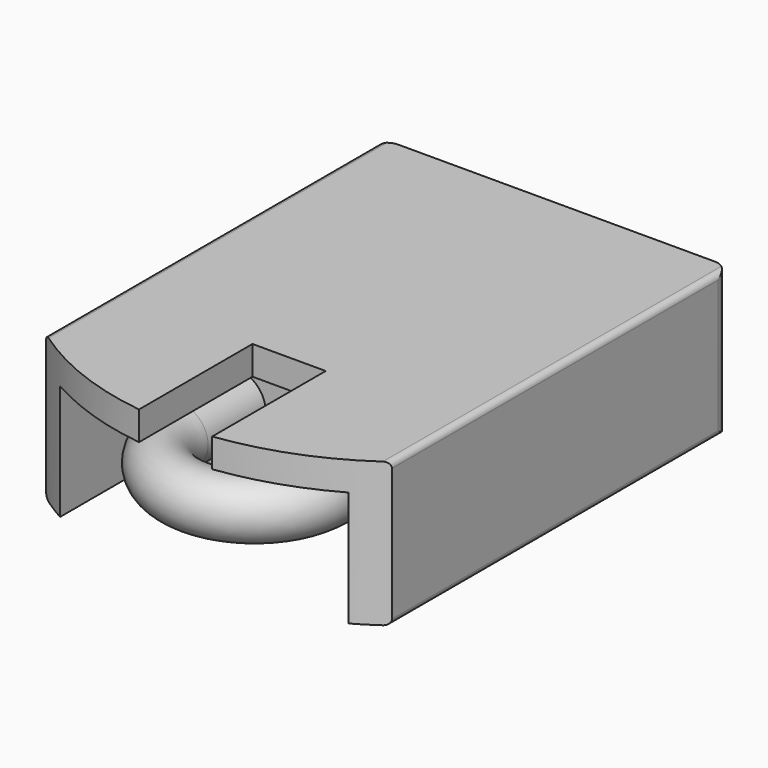
from build123d import *

# Parameters (mm, degrees)
F1_DEPTH    = 25
F3_R        = 2.54
F4_W        = 50
F4_H        = 30
F5_DEPTH    = 20
F2_W        = 12.7
F2_H        = 25
F6_DEPTH    = 25
F7_T1_DEPTH = 75.655609521
F9_W        = 5
F9_H        = 15
F10_DEPTH   = 10
F11_W       = 7.3
F11_H       = 11.5
F12_DEPTH   = 25.4
F15_R       = 4.9651178244


# Not quite as in the source:
# - a fillet or chamfer that OpenCascade refuses, or shapes differently, is made with other operations: its cross-section is extruded or revolved along the edge and cut away or added
# - a feature names something its author has since deleted; it is built from what else it names


with BuildPart() as f1:
    # F0 (on Top) → F1 (new body)
    with BuildSketch(Plane.XY):
        with BuildLine():
            Line((30, -36.5978047605), (30, 36.5978047605))
            Line((30, 36.5978047605), (-30, 36.5978047605))
            Line((-30, 36.5978047605), (-30, -36.5978047605))
            ThreePointArc((-30, -36.5978047605), (0, -46.4021952395), (30, -36.5978047605))
        make_face()
    extrude(amount=F1_DEPTH)

    # F3
    f3_edges = [f1.edges().sort_by_distance(p)[0] for p in [
        (-30, 36.597805, 12.5),
        (30, 36.597805, 12.5),
    ]]
    fillet(f3_edges, radius=F3_R)

    # F4 (on face) → F5 (cut)
    with BuildSketch(Plane.XY):
        with Locations((0, -31.4021952395)):
            Rectangle(F4_W, F4_H)
    extrude(amount=F5_DEPTH, mode=Mode.SUBTRACT)

    # F2 (on Top) → F6 (cut, through all)
    with BuildSketch(Plane.XY):
        with Locations((0, -33.9021952395)):
            Rectangle(F2_W, F2_H)
    extrude(amount=F6_DEPTH, mode=Mode.SUBTRACT)

    # F7: fillet of radius 1 on 4 edges, made by hand

    # F7_s2 → F7_t1 (cut)
    with BuildSketch(Plane.XZ.offset(-36.5578047605)):
        with BuildLine():
            ThreePointArc((29, 0), (29.7071067812, 0.2928932188), (30, 1))
            Line((30, 1), (30, 0))
            Line((30, 0), (29, 0))
        make_face()
        with BuildLine():
            ThreePointArc((29, 25), (29.7071067812, 24.7071067812), (30, 24))
            Line((30, 24), (30, 25))
            Line((30, 25), (29, 25))
        make_face()
        with BuildLine():
            ThreePointArc((-29, 25), (-29.7071067812, 24.7071067812), (-30, 24))
            Line((-30, 24), (-30, 25))
            Line((-30, 25), (-29, 25))
        make_face()
        with BuildLine():
            ThreePointArc((-29, 0), (-29.7071067812, 0.2928932188), (-30, 1))
            Line((-30, 1), (-30, 0))
            Line((-30, 0), (-29, 0))
        make_face()
    extrude(amount=F7_T1_DEPTH, mode=Mode.SUBTRACT)

    # F9 (on face) → F10 (cut)
    with BuildSketch(Plane(origin=(0, 36.5978047605, 0), x_dir=(-1, 0, 0), z_dir=(0, 1, 0))):
        with Locations((-15.5, 12.5)):
            Rectangle(F9_W, F9_H)
        with Locations((15.5, 12.5)):
            Rectangle(F9_W, F9_H)
        with Locations((-5.5, 12.5)):
            Rectangle(F9_W, F9_H)
        with Locations((5.5, 12.5)):
            Rectangle(F9_W, F9_H)
    extrude(amount=-F10_DEPTH, mode=Mode.SUBTRACT)

    # F11 (on face) → F12 (cut)
    with BuildSketch(Plane(origin=(0, 36.5978047605, 0), x_dir=(-1, 0, 0), z_dir=(0, 1, 0))):
        with Locations((23.35, 12.5)):
            Rectangle(F11_W, F11_H)
    extrude(amount=-F12_DEPTH, mode=Mode.SUBTRACT)

    # F16: sweep along a path in F14
    with BuildLine(Plane.XY.offset(12)) as f16_path:
        Line((-13, -16.4021952395), (-13, -28.9021952395))
        ThreePointArc((-13, -28.9021952395), (0, -41.9021952395), (13, -28.9021952395))
        Line((13, -28.9021952395), (13, -16.4021952395))
    # F15 (on face) → F16 (sweep)
    with BuildSketch(Plane.XZ.offset(16.4021952395)):
        with Locations((-12.9998130724, 11.9997570291)):
            Circle(F15_R)
    sweep(path=f16_path.line)


solid = f1.part
